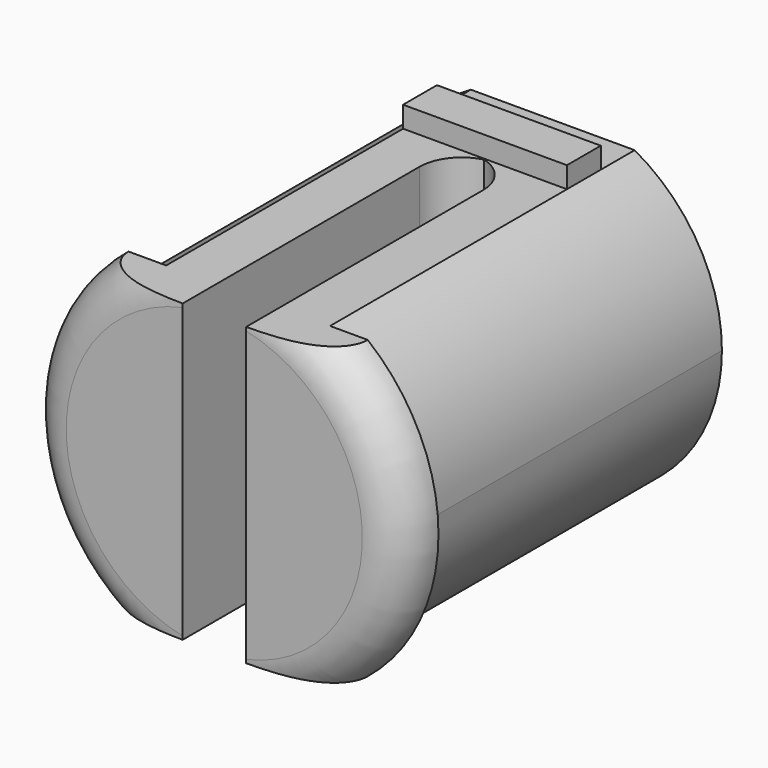
from build123d import *

# Parameters (mm, degrees)
F1_DEPTH    = 10
F3_DEPTH    = 1
F2_W        = 1.5
F2_H        = 7
F4_DEPTH    = 8
F6_T1_DEPTH = 7
F6_T4_ANGLE = 165.8100193305
F6_T6_ANGLE = 165.8100193305
F7_DEPTH    = 0.5


# Not quite as in the source:
# - a fillet or chamfer that OpenCascade refuses, or shapes differently, is made with other operations: its cross-section is extruded or revolved along the edge and cut away or added


with BuildPart() as f1:
    # F0 (on Front) → F1 (new body)
    with BuildSketch(Plane.XZ):
        with BuildLine():
            ThreePointArc((1.9364916731, -3.5), (3.4457195687, -2.0315060063), (4, 0))
            ThreePointArc((4, 0), (3.4457195687, 2.0315060063), (1.9364916731, 3.5))
            Line((1.9364916731, 3.5), (-1.9364916731, 3.5))
            ThreePointArc((-1.9364916731, 3.5), (-4, 0), (-1.9364916731, -3.5))
            Line((-1.9364916731, -3.5), (1.9364916731, -3.5))
        make_face()
    extrude(amount=F1_DEPTH)

    # F2 (on face) → F3 (join)
    with BuildSketch(Plane.XZ.offset(10)):
        with BuildLine():
            Line((-1.9364916731, 3.5), (-2.8284271247, 3.5))
            ThreePointArc((-2.8284271247, 3.5), (-4.5, 0), (-2.8284271247, -3.5))
            Line((-2.8284271247, -3.5), (-1.9364916731, -3.5))
            ThreePointArc((-1.9364916731, -3.5), (-4, 0), (-1.9364916731, 3.5))
        make_face()
        with BuildLine():
            ThreePointArc((2.8284271247, -3.5), (4.0606601718, -1.9393398282), (4.5, 0))
            ThreePointArc((4.5, 0), (4.0606601718, 1.9393398282), (2.8284271247, 3.5))
            Line((2.8284271247, 3.5), (1.9364916731, 3.5))
            ThreePointArc((1.9364916731, 3.5), (4, 0), (1.9364916731, -3.5))
            Line((1.9364916731, -3.5), (2.8284271247, -3.5))
        make_face()
    extrude(amount=-F3_DEPTH)

    # F2 (on face) → F4 (cut)
    with BuildSketch(Plane.XZ.offset(10)):
        Rectangle(F2_W, F2_H)
    extrude(amount=-F4_DEPTH, mode=Mode.SUBTRACT)

    # F6: fillet of radius 1 on 4 edges, made by hand

    # F6_s2 → F6_t1 (join)
    with BuildSketch(Plane.XY.offset(-3.5)):
        with BuildLine():
            ThreePointArc((0.25, -2), (-0.4571067812, -2.2928932188), (-0.75, -3))
            Line((-0.75, -3), (-0.75, -2))
            Line((-0.75, -2), (0.25, -2))
        make_face()
        with BuildLine():
            ThreePointArc((0.75, -3), (0.4571067812, -2.2928932188), (-0.25, -2))
            Line((-0.25, -2), (0.75, -2))
            Line((0.75, -2), (0.75, -3))
        make_face()
    extrude(amount=F6_T1_DEPTH)

    # F6_s3 → F6_t4 (revolve, cut)
    with BuildSketch(Plane(origin=(0, 0, 0), x_dir=(0, 1, 0), z_dir=(0.9923427412, 0, 0.1235147116))):
        with BuildLine():
            ThreePointArc((-10, 3.5), (-9.7071067812, 4.2071067812), (-9, 4.5))
            Line((-9, 4.5), (-10, 4.5))
            Line((-10, 4.5), (-10, 3.5))
        make_face()
    revolve(axis=Axis((0, -10, 0), (0, -1, 0)), revolution_arc=F6_T4_ANGLE, mode=Mode.SUBTRACT)

    # F6_s5 → F6_t6 (revolve, cut)
    with BuildSketch(Plane(origin=(0, 0, 0), x_dir=(0, 1, 0), z_dir=(-0.9923427412, 0, -0.1235147116))):
        with BuildLine():
            ThreePointArc((-9, 4.5), (-9.7071067812, 4.2071067812), (-10, 3.5))
            Line((-10, 3.5), (-10, 4.5))
            Line((-10, 4.5), (-9, 4.5))
        make_face()
    revolve(axis=Axis((0, -10, 0), (0, -1, 0)), revolution_arc=F6_T6_ANGLE, mode=Mode.SUBTRACT)

    # F5 (on face) → F7 (join)
    with BuildSketch(Plane.XY.offset(3.5)):
        Polygon((-1.9364916731, -1), (-1.9364916731, -2), (-0.75, -2), (0.75, -2), (1.9364916731, -2), (1.9364916731, -1), align=None)
    extrude(amount=F7_DEPTH)


solid = f1.part
